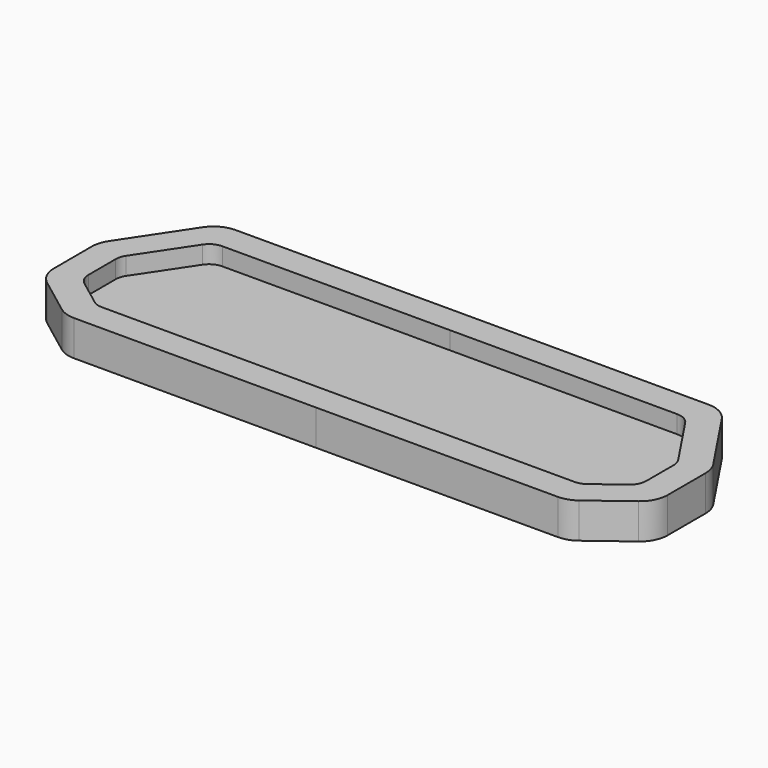
from build123d import *

# Parameters (mm, degrees)
F1_DEPTH = 6.35
F2_DEPTH = 3.175
F3_R     = 5
F4_R     = 3


# Not quite as in the source:
# - ends of sketch curves that miss each other by under 0.0002 mm in the source are joined
# - a feature names something its author has since deleted; it is built from what else it names


with BuildPart() as f1:
    # F0 (on Top) → F1 (new body)
    with BuildSketch(Plane.XY):
        Polygon((0, 12.50001), (0, 17.5), (-0.0375035219, 17.5), (-45.0252224641, 17.4621137515), (-54.9730516553, 2.5016534816), (-54.9460702886, -9.9983173986), (-45.0221895285, -17.4832638625), (-0.0259340823, -17.4999907076), (0, -17.5), (0, -12.50001), (-43.3485360617, -12.4839008237), (-49.9514424363, -7.508736751), (-49.9698707033, 1.0287403501), (-42.3475575474, 12.4643751943), align=None)
        Polygon((54.9832946886, 2.5222222222), (45, 17.5), (0, 17.5), (0, 12.50001), (42.3238055081, 12.50001), (49.9833046886, 1.0085855561), (49.9833046886, -7.4847291513), (43.3271563883, -12.50001), (0, -12.50001), (0, -17.5), (45, -17.5), (54.9832946886, -9.9777777778), align=None)
    extrude(amount=F1_DEPTH)

    # F0 (on Top) → F2 (join)
    with BuildSketch(Plane.XY):
        Polygon((0, -12.50001), (0, 12.50001), (-42.3475575474, 12.4643751943), (-49.9698707033, 1.0287403501), (-49.9514424363, -7.508736751), (-43.3485360617, -12.4839008237), align=None)
        Polygon((42.3238055081, 12.50001), (0, 12.50001), (0, -12.50001), (43.3271563883, -12.50001), (49.9833046886, -7.4847291513), (49.9833046886, 1.0085855561), align=None)
    extrude(amount=F2_DEPTH)

    # F3
    f3_edges = [f1.edges().sort_by_distance(p)[0] for p in [
        (-45.02219, -17.483264, 3.175),
        (-45.025222, 17.462114, 3.175),
        (45, 17.5, 3.175),
        (54.983295, 2.522222, 3.175),
        (54.983295, -9.977778, 3.175),
        (45, -17.5, 3.175),
        (-54.973052, 2.501653, 3.175),
        (-54.94607, -9.998317, 3.175),
    ]]
    fillet(f3_edges, radius=F3_R)

    # F4
    f4_edges = [f1.edges().sort_by_distance(p)[0] for p in [
        (-42.347558, 12.464375, 4.7625),
        (-49.969871, 1.02874, 4.7625),
        (-49.951442, -7.508737, 4.7625),
        (-43.348536, -12.483901, 4.7625),
        (43.327156, -12.50001, 4.7625),
        (49.983305, -7.484729, 4.7625),
        (49.983305, 1.008586, 4.7625),
        (42.323806, 12.50001, 4.7625),
    ]]
    fillet(f4_edges, radius=F4_R)


solid = f1.part
